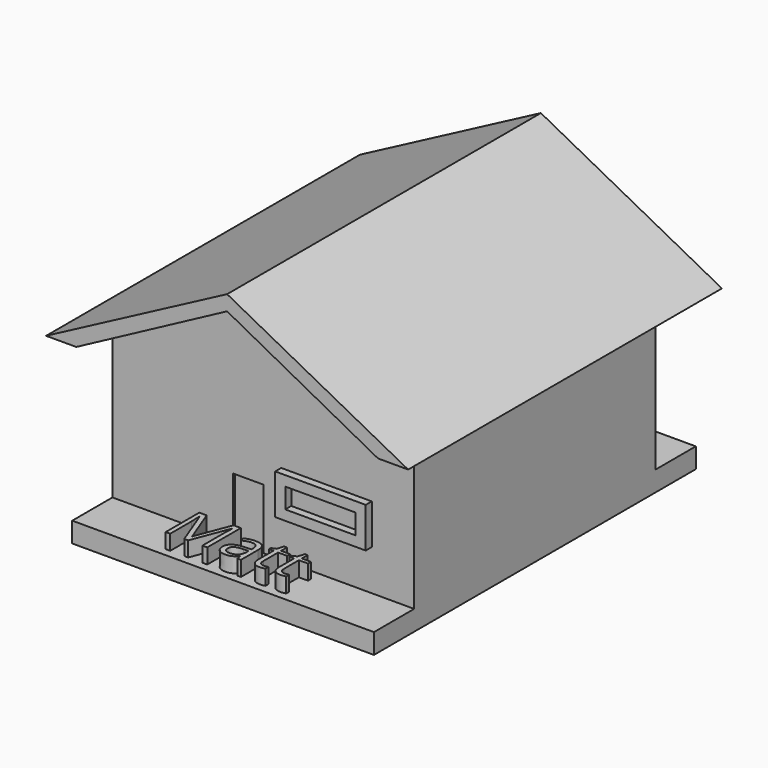
from build123d import *

# Parameters (mm, degrees)
F1_DEPTH     = 5943.6
F2_DEPTH     = 4572
F0_W         = 2743.2
F0_H         = 1219.2
F3_DEPTH     = 4572
F0_W_2       = 914.4
F0_H_2       = 1828.8
F4_DEPTH     = 4495.8
F0_W_3       = 2133.6
F0_H_3       = 609.6
F5_DEPTH     = 4800.6
F6_DEPTH     = 4572
F7_DEPTH     = 6096
F8_TEXT_SIZE = 1782.5213114421
F9_DEPTH     = 457.2


# Not quite as in the source:
# - Text() gives the source's letters only with a copy of the font that has no kerning and outlines rounded to 1/6400 em; it was checked with that copy


with BuildPart() as f1:
    # F0 (on Front) → F1 (new body, symmetric)
    with BuildSketch(Plane.XZ):
        Polygon((-5486.4, 4572), (-4572, 4572), (0, 7010.4), (0, 7467.6), align=None)
        Polygon((0, 7010.4), (4572, 4572), (5486.4, 4572), (0, 7467.6), align=None)
    extrude(amount=F1_DEPTH, both=True)

    # F0 (on Front) → F2 (join, symmetric)
    with BuildSketch(Plane.XZ):
        Polygon((-4572, 4572), (4572, 4572), (0, 7010.4), align=None)
    extrude(amount=F2_DEPTH, both=True)

    # F0 (on Front) → F3 (join, symmetric)
    with BuildSketch(Plane.XZ):
        Polygon((0, 1828.8), (0, 0), (4572, 0), (4572, 4572), (-4572, 4572), (-4572, 0), (-914.4, 0), (-914.4, 1828.8), align=None)
        with Locations((1914.9912277222, 1840.7087511063)):
            Rectangle(F0_W, F0_H, mode=Mode.SUBTRACT)
    extrude(amount=F3_DEPTH, both=True)

    # F0 (on Front) → F4 (join, symmetric)
    with BuildSketch(Plane.XZ):
        with Locations((-457.2, 914.4)):
            Rectangle(F0_W_2, F0_H_2)
    extrude(amount=F4_DEPTH, both=True)

    # F0 (on Front) → F5 (join, symmetric)
    with BuildSketch(Plane.XZ):
        with Locations((1914.9912277222, 1840.7087511063)):
            Rectangle(F0_W, F0_H)
        with Locations((1914.9912277222, 1840.7087511063)):
            Rectangle(F0_W_3, F0_H_3, mode=Mode.SUBTRACT)
    extrude(amount=F5_DEPTH, both=True)

    # F0 (on Front) → F6 (join, symmetric)
    with BuildSketch(Plane.XZ):
        with Locations((1914.9912277222, 1840.7087511063)):
            Rectangle(F0_W_3, F0_H_3)
    extrude(amount=F6_DEPTH, both=True)

    # F0 (on Front) → F7 (join, symmetric)
    with BuildSketch(Plane.XZ):
        Polygon((4572, 0), (0, 0), (-914.4, 0), (-4572, 0), (-4572, -609.6), (4572, -609.6), align=None)
    extrude(amount=F7_DEPTH, both=True)

    # F8 (on face) → F9 (join, symmetric)
    with BuildSketch(Plane.XY):
        with Locations((-2107.0210933685, -5855.4153442383)):
            Text('Matt', F8_TEXT_SIZE, font='Open Sans', text_align=(TextAlign.LEFT, TextAlign.BOTTOM))
    extrude(amount=F9_DEPTH, both=True)


solid = f1.part
